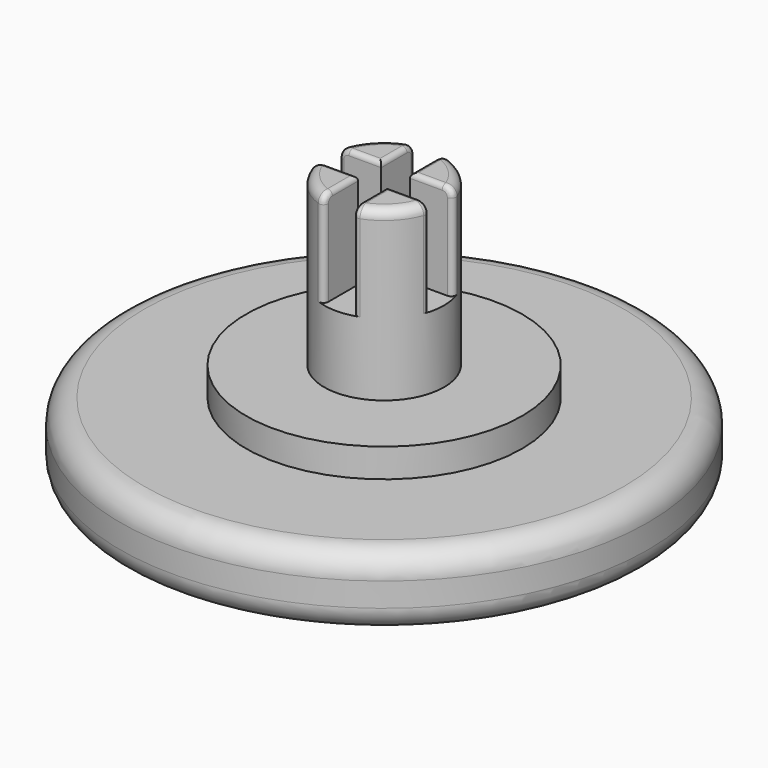
from build123d import *

# Parameters (mm, degrees)
F0_R      = 11
F1_DEPTH  = 3
F2_R      = 5.75
F3_DEPTH  = 1.2
F4_R      = 2.5
F5_DEPTH  = 7
F6_R      = 0.6
F10_DEPTH = 7
F11_W     = 1.2
F11_H     = 2.8315826069
F11_H_2   = 1.2
F11_W_2   = 2.9928033758
F12_DEPTH = 4
F13_R     = 0.4
F14_R     = 1
F15_R     = 0.2


# Not quite as in the source:
# - a feature of the source that left no trace in its solid (it failed there, or was rolled back) is left out


with BuildPart() as f1:
    # F0 (on Top) → F1 (new body)
    with BuildSketch(Plane.XY):
        Circle(F0_R)
    extrude(amount=F1_DEPTH)

    # F2 (on face) → F3 (join)
    with BuildSketch(Plane.XY.offset(3)):
        Circle(F2_R)
    extrude(amount=F3_DEPTH)

    # F4 (on face) → F5 (join)
    with BuildSketch(Plane.XY.offset(4.2)):
        Circle(F4_R)
    extrude(amount=F5_DEPTH)

    # F6 (on face) → F10 (cut)
    with BuildSketch(Plane.XY.offset(11.2)):
        Circle(F6_R)
    extrude(amount=-F10_DEPTH, mode=Mode.SUBTRACT)

    # F11 (on face) → F12 (cut)
    with BuildSketch(Plane.XY.offset(11.2)):
        with Locations((0, 2.0157913034)):
            Rectangle(F11_W, F11_H)
        Rectangle(F11_W, F11_H_2)
        with Locations((-2.0964016879, 0)):
            Rectangle(F11_W_2, F11_H_2)
        with Locations((2.0964016879, 0)):
            Rectangle(F11_W_2, F11_H_2)
        with Locations((0, -2.0157913034)):
            Rectangle(F11_W, F11_H)
    extrude(amount=-F12_DEPTH, mode=Mode.SUBTRACT)

    # F13
    f13_edges = [f1.edges().sort_by_distance(p)[0] for p in [
        (1.767767, -1.767767, 11.2),
        (-1.767767, -1.767767, 11.2),
        (-1.767767, 1.767767, 11.2),
        (1.767767, 1.767767, 11.2),
    ]]
    fillet(f13_edges, radius=F13_R)

    # F14
    f14_edges = [f1.edges().sort_by_distance(p)[0] for p in [
        (-11, 0, 3),
        (-11, 0, 0),
    ]]
    fillet(f14_edges, radius=F14_R)

    # F15
    f15_edges = [f1.edges().sort_by_distance(p)[0] for p in [
        (-0.6, 1.306231, 11.2),
        (-1.484924, 1.484924, 11.2),
        (-1.306231, 0.6, 11.2),
        (1.306231, 0.6, 11.2),
        (1.484924, 1.484924, 11.2),
        (0.6, 1.306231, 11.2),
        (0.6, -1.306231, 11.2),
        (1.484924, -1.484924, 11.2),
        (1.306231, -0.6, 11.2),
        (-1.306231, -0.6, 11.2),
        (-1.484924, -1.484924, 11.2),
        (-0.6, -1.306231, 11.2),
        (-0.6, 0, 7.2),
        (2.426932, -0.6, 9),
        (0.6, -2.426932, 9),
        (-0.6, -2.426932, 9),
        (-2.426932, -0.6, 9),
        (2.426932, 0.6, 9),
        (-2.426932, 0.6, 9),
        (0.6, 2.426932, 9),
        (-0.6, 2.426932, 9),
        (2.305572, -0.6, 11.08332),
        (0.6, -2.305572, 11.08332),
        (-0.6, -2.305572, 11.08332),
        (-2.305572, -0.6, 11.08332),
        (2.305572, 0.6, 11.08332),
        (0.6, 2.305572, 11.08332),
        (-2.305572, 0.6, 11.08332),
        (-0.6, 2.305572, 11.08332),
    ]]
    fillet(f15_edges, radius=F15_R)


solid = f1.part
